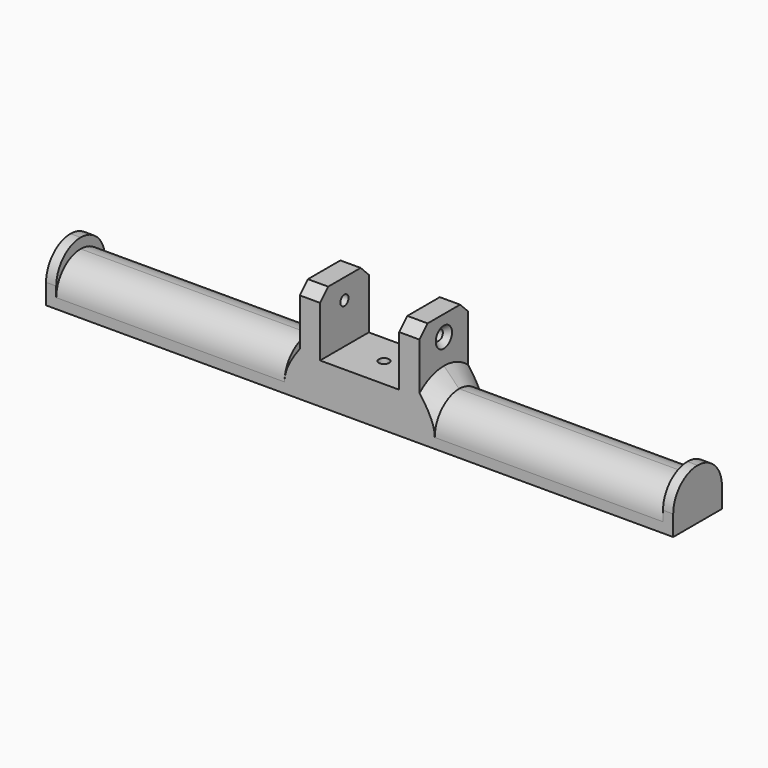
from build123d import *

# Parameters (mm, degrees)
F1_DEPTH     = 30
F2_R         = 14.99999
F4_DEPTH     = 299.001
F5_T1_DEPTH  = 2e-05
F5_T6_ANGLE  = 163.702935025
F5_T12_ANGLE = 163.702935025
F5_T18_ANGLE = 163.702935025
F5_T24_ANGLE = 163.702935025
F6_SIZE      = 5
F7_R         = 2.5
F8_DEPTH     = 179.001
F9_W         = 20
F9_H         = 20
F11_R        = 2.5
F12_DEPTH    = 20.001
F13_SIZE     = 2.5
F14_W        = 5
F14_H        = 25
F15_DEPTH    = 30
F16_R        = 14.99999
F17_R        = 5
F18_DEPTH    = 7.5
F19_SIZE     = 2.49999


# Not quite as in the source:
# - a fillet or chamfer that OpenCascade refuses, or shapes differently, is made with other operations: its cross-section is extruded or revolved along the edge and cut away or added
# - a fillet or chamfer is up to 0.001 mm smaller than in the source, because OpenCascade refuses the exact size


with BuildPart() as f1:
    # F0 (on Front) → F1 (new body)
    with BuildSketch(Plane.XZ):
        Polygon((-149.5, 0), (0, 0), (149.5, 0), (149.5, 20), (29.5, 20), (29.5, 50), (19.5, 50), (19.5, 20), (0, 20), (-19.5, 20), (-19.5, 50), (-29.5, 50), (-29.5, 20), (-149.5, 20), align=None)
    extrude(amount=F1_DEPTH)

    # F2 (radius 15 in the source; OpenCascade refuses exactly that, so slightly less here)
    f2_edges = [f1.edges().sort_by_distance(p)[0] for p in [
        (-89.5, 0, 20),
        (-89.5, -30, 20),
        (89.5, 0, 20),
        (89.5, -30, 20),
    ]]
    fillet(f2_edges, radius=F2_R)

    # F3 (on face) → F4 (cut, through all)
    with BuildSketch(Plane(origin=(-149.5, 0, 0), x_dir=(0, -1, 0), z_dir=(-1, 0, 0))):
        with BuildLine():
            Line((25, 0), (25, 5))
            ThreePointArc((25, 5), (15, 15), (5, 5))
            Line((5, 5), (5, 0))
            Line((5, 0), (25, 0))
        make_face()
    extrude(amount=-F4_DEPTH, mode=Mode.SUBTRACT)

    # F5: chamfer of 7.5 on 4 edges, made by hand

    # F5_s2 → F5_t1 (join)
    with BuildSketch(Plane.XZ.offset(14.99999)):
        Polygon((-37, 20), (-29.5, 27.5), (-29.5, 20), align=None)
        Polygon((37, 20), (29.5, 27.5), (29.5, 20), align=None)
    extrude(amount=F5_T1_DEPTH)


with BuildPart() as f5_tool4:
    # F5_s5 → F5_t6 (revolve)
    with BuildSketch(Plane(origin=(0, -12.4720838446, -3.6463990318), x_dir=(1, 0, 0), z_dir=(0, -0.9598196681, -0.2806175417))):
        Polygon((-37, -5.9916217418), (-29.5, -13.4916217418), (-29.5, -5.9916217418), align=None)
    revolve(axis=Axis((-29.5, -14.99999, 5.00001), (1, 0, 0)), revolution_arc=F5_T6_ANGLE)

    split(bisect_by=Plane.XZ, keep=Keep.TOP)

    split(bisect_by=Plane.XY, keep=Keep.TOP)


with BuildPart() as f1_1:
    add(f1.part)

    # F5_t3: union F5_tool4
    add(f5_tool4.part)


with BuildPart() as f5_tool10:
    # F5_s11 → F5_t12 (revolve)
    with BuildSketch(Plane(origin=(0, -12.4720838446, -3.6463990318), x_dir=(1, 0, 0), z_dir=(0, -0.9598196681, -0.2806175417))):
        Polygon((29.5, -13.4916217418), (37, -5.9916217418), (29.5, -5.9916217418), align=None)
    revolve(axis=Axis((29.5, -14.99999, 5.00001), (1, 0, 0)), revolution_arc=F5_T12_ANGLE)

    split(bisect_by=Plane.XZ, keep=Keep.TOP)

    split(bisect_by=Plane.XY, keep=Keep.TOP)


with BuildPart() as f1_2:
    add(f1_1.part)

    # F5_t9: union F5_tool10
    add(f5_tool10.part)


with BuildPart() as f5_tool16:
    # F5_s17 → F5_t18 (revolve)
    with BuildSketch(Plane.XZ.offset(15.00001)):
        Polygon((37, 20), (29.5, 27.5), (29.5, 20), align=None)
    revolve(axis=Axis((29.5, -15.00001, 5.00001), (1, 0, 0)), revolution_arc=F5_T18_ANGLE)

    split(bisect_by=Plane.XY, keep=Keep.TOP)

    split(bisect_by=Plane.XZ.offset(30), keep=Keep.BOTTOM)


with BuildPart() as f1_3:
    add(f1_2.part)

    # F5_t15: union F5_tool16
    add(f5_tool16.part)


with BuildPart() as f5_tool22:
    # F5_s23 → F5_t24 (revolve)
    with BuildSketch(Plane.XZ.offset(15.00001)):
        Polygon((-37, 20), (-29.5, 27.5), (-29.5, 20), align=None)
    revolve(axis=Axis((-29.5, -15.00001, 5.00001), (1, 0, 0)), revolution_arc=F5_T24_ANGLE)

    split(bisect_by=Plane.XY, keep=Keep.TOP)

    split(bisect_by=Plane.XZ.offset(30), keep=Keep.BOTTOM)


with BuildPart() as f1_4:
    add(f1_3.part)

    # F5_t21: union F5_tool22
    add(f5_tool22.part)

    # F6
    f6_edges = [f1_4.edges().sort_by_distance(p)[0] for p in [
        (-24.5, 0, 50),
        (-24.5, -30, 50),
        (24.5, 0, 50),
        (24.5, -30, 50),
    ]]
    chamfer(f6_edges, length=F6_SIZE)

    # F7 (on face) → F8 (cut, through all)
    with BuildSketch(Plane.YZ.offset(29.5)):
        with Locations((-15, 40)):
            Circle(F7_R)
    extrude(amount=-F8_DEPTH, mode=Mode.SUBTRACT)

    # F9 (on face) → F10 (join, up to the next surface of F1)
    with BuildSketch(Plane(origin=(0, 0, 0), x_dir=(1, 0, 0), z_dir=(0, 0, -1))):
        with Locations((0, 15)):
            Rectangle(F9_W, F9_H)
    extrude(until=Until.NEXT, dir=(0, 0, 1))

    # F11 (on face) → F12 (cut, through all)
    with BuildSketch(Plane.XY.offset(20)):
        with Locations((0, -15)):
            Circle(F11_R)
    extrude(amount=-F12_DEPTH, mode=Mode.SUBTRACT)

    # F13
    f13_edges = [f1_4.edges().sort_by_distance(p)[0] for p in [
        (-29.5, -17.5, 40),
        (29.5, -17.5, 40),
    ]]
    chamfer(f13_edges, length=F13_SIZE)

    # F14 (on face) → F15 (join, through all)
    with BuildSketch(Plane.XZ.offset(30)):
        with Locations((-152, 12.5)):
            Rectangle(F14_W, F14_H)
        with Locations((152, 12.5)):
            Rectangle(F14_W, F14_H)
    extrude(amount=-F15_DEPTH)

    # F16 (radius 15 in the source; OpenCascade refuses exactly that, so slightly less here)
    f16_edges = [f1_4.edges().sort_by_distance(p)[0] for p in [
        (152, 0, 25),
        (152, -30, 25),
        (-152, -30, 25),
        (-152, 0, 25),
    ]]
    fillet(f16_edges, radius=F16_R)

    # F17 (on face) → F18 (cut)
    with BuildSketch(Plane(origin=(0, 0, 0), x_dir=(1, 0, 0), z_dir=(0, 0, -1))):
        with Locations((0, 15)):
            Circle(F17_R)
    extrude(amount=-F18_DEPTH, mode=Mode.SUBTRACT)

    # F19 (size 2.5 in the source; OpenCascade refuses exactly that, so slightly less here)
    f19_edges = [f1_4.edges().sort_by_distance(p)[0] for p in [
        (-2.5, -15, 7.5),
    ]]
    chamfer(f19_edges, length=F19_SIZE)


solid = f1_4.part
